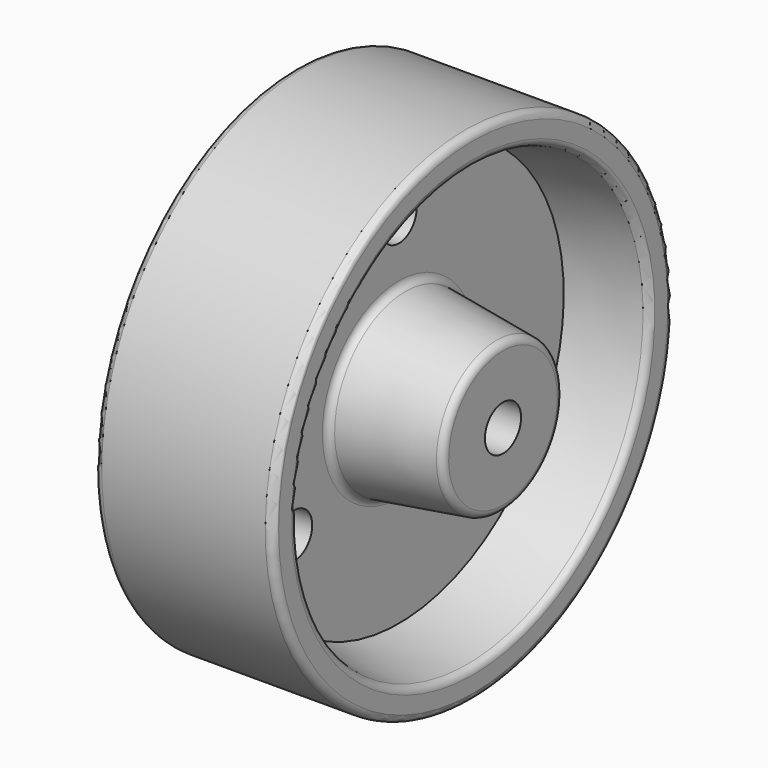
from build123d import *

# Parameters (mm, degrees)
F2_R     = 4.826
F2_R_2   = 1.5875
F3_DEPTH = 50.8010001
F4_R     = 4.7625
F5_DEPTH = 28.5760001


with BuildPart() as f1:
    # F0 (on Front) → F1 (revolve)
    with BuildSketch(Plane.XZ):
        Polygon((0.4836565733, 28.1133555889), (-5.8663434267, 28.1133555889), (-5.8663434267, 20.1758555889), (-2.6913434267, 20.1758555889), (0.4836565733, 20.1758555889), align=None)
        with BuildLine():
            Line((0.4836565733, 10.6508555889), (-5.8663434267, 10.6508555889))
            Line((-5.8663434267, 10.6508555889), (-5.8663434267, 4.5518314502))
            ThreePointArc((-5.8663434267, 4.5518314502), (-6.2545602731, 3.5116986858), (-7.2293370237, 2.980286629))
            Line((-7.2293370237, 2.980286629), (-26.7283498297, 0.194713371))
            ThreePointArc((-26.7283498297, 0.194713371), (-27.7031265803, -0.3366986858), (-28.0913434267, -1.3768314502))
            Line((-28.0913434267, -1.3768314502), (-28.0913434267, -14.2875))
            ThreePointArc((-28.0913434267, -14.2875), (-27.6263754418, -15.4100320151), (-26.5038434267, -15.875))
            Line((-26.5038434267, -15.875), (21.1211565733, -15.875))
            ThreePointArc((21.1211565733, -15.875), (22.2436885884, -15.4100320151), (22.7086565733, -14.2875))
            Line((22.7086565733, -14.2875), (22.7086565733, -1.3768314502))
            ThreePointArc((22.7086565733, -1.3768314502), (22.3204397269, -0.3366986858), (21.3456629763, 0.194713371))
            Line((21.3456629763, 0.194713371), (1.8466501703, 2.980286629))
            ThreePointArc((1.8466501703, 2.980286629), (0.8718734197, 3.5116986858), (0.4836565733, 4.5518314502))
            Line((0.4836565733, 4.5518314502), (0.4836565733, 10.6508555889))
        make_face()
        Polygon((-2.6913434267, 20.1758555889), (-5.8663434267, 20.1758555889), (-5.8663434267, 10.6508555889), (0.4836565733, 10.6508555889), (0.4836565733, 20.1758555889), align=None)
        with BuildLine():
            Line((14.7711565733, 37.6383555889), (-20.1538434267, 37.6383555889))
            ThreePointArc((-20.1538434267, 37.6383555889), (-21.2763754418, 37.173387604), (-21.7413434267, 36.0508555889))
            Line((-21.7413434267, 36.0508555889), (-21.7413434267, 32.5897942845))
            ThreePointArc((-21.7413434267, 32.5897942845), (-21.3815240761, 31.5833368968), (-20.4651777912, 31.0331224618))
            Line((-20.4651777912, 31.0331224618), (-5.8663434267, 28.1133555889))
            Line((-5.8663434267, 28.1133555889), (0.4836565733, 28.1133555889))
            Line((0.4836565733, 28.1133555889), (15.0824909378, 31.0331224618))
            ThreePointArc((15.0824909378, 31.0331224618), (15.9988372227, 31.5833368968), (16.3586565733, 32.5897942845))
            Line((16.3586565733, 32.5897942845), (16.3586565733, 36.0508555889))
            ThreePointArc((16.3586565733, 36.0508555889), (15.8936885884, 37.173387604), (14.7711565733, 37.6383555889))
        make_face()
    revolve(axis=Axis((-2.6913434267, 0, -15.875), (-1, 0, 0)))

    # F2 (on face) → F3 (cut, through all)
    with BuildSketch(Plane(origin=(-28.0913434267, 0, 0), x_dir=(0, -1, 0), z_dir=(-1, 0, 0))):
        with Locations((0, -15.875)):
            Circle(F2_R)
        with Locations((0, -15.875)):
            Circle(F2_R_2, mode=Mode.SUBTRACT)
        with Locations((0, -15.875)):
            Circle(F2_R_2)
    extrude(amount=-F3_DEPTH, mode=Mode.SUBTRACT)

    # F4 (on face) → F5 (cut, through all)
    with BuildSketch(Plane(origin=(-5.8663434267, 0, 0), x_dir=(0, -1, 0), z_dir=(-1, 0, 0))):
        with BuildLine():
            ThreePointArc((0, 11.5847946733), (3.3675960454, 12.9796986279), (4.7625, 16.3472946733))
            ThreePointArc((4.7625, 16.3472946733), (-3.3675960454, 19.7148907187), (0, 11.5847946733))
        make_face()
        with Locations((27.8988178469, -31.982389994)):
            Circle(F4_R)
        with Locations((-27.8886323176, -31.9765093759)):
            Circle(F4_R)
    extrude(amount=-F5_DEPTH, mode=Mode.SUBTRACT)


solid = f1.part
